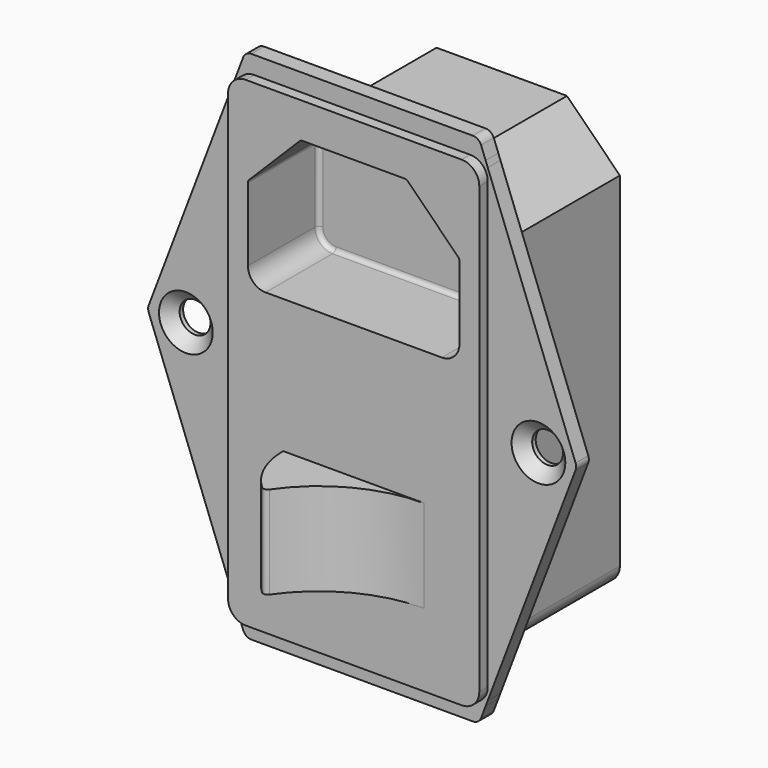
from build123d import *

# Parameters (mm, degrees)
F0_W          = 26.8
F0_H          = 47
F1_DEPTH      = 18
F2_SIZE       = 6
F3_R          = 2
F5_DEPTH      = 5
F6_R          = 1
F7_W          = 28.5
F7_H          = 54.5
F8_DEPTH      = 3
F10_R         = 1.75
F11_DEPTH     = 1.8
F12_T4_DEPTH  = 13
F12_T9_DEPTH  = 13
F12_T14_DEPTH = 13
F12_T19_DEPTH = 13
F12_T24_DEPTH = 13
F12_T29_DEPTH = 13
F12_T34_DEPTH = 13
F12_T39_DEPTH = 13
F13_R         = 1
F14_SIZE      = 1.3
F15_W         = 24
F15_H         = 16.5
F16_DEPTH     = 10
F17_SIZE      = 6
F19_R         = 2
F20_R         = 0.5
F21_W         = 16
F21_H         = 10.5
F22_DEPTH     = 10
F24_DEPTH     = 10.5
F25_R         = 0.5


# Not quite as in the source:
# - a fillet or chamfer that OpenCascade refuses, or shapes differently, is made with other operations: its cross-section is extruded or revolved along the edge and cut away or added


with BuildPart() as f1:
    # F0 (on Front) → F1 (new body)
    with BuildSketch(Plane.XZ):
        Rectangle(F0_W, F0_H)
    extrude(amount=-F1_DEPTH)

    # F2
    f2_edges = [f1.edges().sort_by_distance(p)[0] for p in [
        (-13.4, 9, 23.5),
        (13.4, 9, 23.5),
    ]]
    chamfer(f2_edges, length=F2_SIZE)

    # F3
    f3_edges = [f1.edges().sort_by_distance(p)[0] for p in [
        (-13.4, 9, -23.5),
        (13.4, 9, -23.5),
    ]]
    fillet(f3_edges, radius=F3_R)

    # F4 (on face) → F5 (cut)
    with BuildSketch(Plane(origin=(0, 18, 0), x_dir=(-1, 0, 0), z_dir=(0, 1, 0))):
        Polygon((-6.5715728753, 21.5), (-11.4, 16.6715728753), (-11.4, -21.5), (11.4, -21.5), (11.4, 16.6715728753), (6.5715728753, 21.5), align=None)
    extrude(amount=-F5_DEPTH, mode=Mode.SUBTRACT)

    # F6
    f6_edges = [f1.edges().sort_by_distance(p)[0] for p in [
        (-11.4, 15.5, -21.5),
        (-11.4, 15.5, 16.671573),
        (-6.571573, 15.5, 21.5),
        (6.571573, 15.5, 21.5),
        (11.4, 15.5, 16.671573),
        (11.4, 15.5, -21.5),
        (-8.985786, 13, 19.085786),
        (0, 13, 21.5),
        (8.985786, 13, 19.085786),
        (11.4, 13, -2.414214),
        (0, 13, -21.5),
        (-11.4, 13, -2.414214),
    ]]
    fillet(f6_edges, radius=F6_R)

    # F7 (on face) → F8 (join)
    with BuildSketch(Plane.XZ):
        Rectangle(F7_W, F7_H)
    extrude(amount=F8_DEPTH)

    # F10 (on offset) → F11 (join)
    with BuildSketch(Plane.XZ.offset(1.8)):
        Polygon((24.35, 0), (13.25, 29.25), (-13.25, 29.25), (-24.35, 0), (-13.25, -29.25), (13.25, -29.25), align=None)
        with Locations((-20, 0)):
            Circle(F10_R, mode=Mode.SUBTRACT)
        with Locations((20, 0)):
            Circle(F10_R, mode=Mode.SUBTRACT)
    extrude(amount=-F11_DEPTH)

    # F12: fillet of radius 2 on 4 edges, made by hand


with BuildPart() as f12_tool2:
    # F12_s3 → F12_t4 (new body)
    with BuildSketch(Plane.XZ.offset(-5)):
        with BuildLine():
            ThreePointArc((12.25, 27.25), (13.6642135624, 26.6642135624), (14.25, 25.25))
            Line((14.25, 25.25), (14.25, 27.25))
            Line((14.25, 27.25), (12.25, 27.25))
        make_face()
    extrude(amount=F12_T4_DEPTH)

    split(bisect_by=Plane.XZ.offset(1.8), keep=Keep.TOP)


with BuildPart() as f1_1:
    add(f1.part)

    # F12_t1: cut F12_tool2
    add(f12_tool2.part, mode=Mode.SUBTRACT)


with BuildPart() as f12_tool7:
    # F12_s8 → F12_t9 (new body)
    with BuildSketch(Plane.XZ.offset(-5)):
        with BuildLine():
            ThreePointArc((12.25, 27.25), (13.6642135624, 26.6642135624), (14.25, 25.25))
            Line((14.25, 25.25), (14.25, 27.25))
            Line((14.25, 27.25), (12.25, 27.25))
        make_face()
    extrude(amount=F12_T9_DEPTH)

    split(bisect_by=Plane(origin=(21.2847693156, 0, 8.0772970736), x_dir=(0, 1, 0), z_dir=(0.9349426915, 0, 0.354798765)), keep=Keep.TOP)


with BuildPart() as f1_2:
    add(f1_1.part)

    # F12_t6: cut F12_tool7
    add(f12_tool7.part, mode=Mode.SUBTRACT)


with BuildPart() as f12_tool12:
    # F12_s13 → F12_t14 (new body)
    with BuildSketch(Plane.XZ.offset(-5)):
        with BuildLine():
            ThreePointArc((-12.25, 27.25), (-13.6642135624, 26.6642135624), (-14.25, 25.25))
            Line((-14.25, 25.25), (-14.25, 27.25))
            Line((-14.25, 27.25), (-12.25, 27.25))
        make_face()
    extrude(amount=F12_T14_DEPTH)

    split(bisect_by=Plane.XZ.offset(1.8), keep=Keep.TOP)


with BuildPart() as f1_3:
    add(f1_2.part)

    # F12_t11: cut F12_tool12
    add(f12_tool12.part, mode=Mode.SUBTRACT)


with BuildPart() as f12_tool17:
    # F12_s18 → F12_t19 (new body)
    with BuildSketch(Plane.XZ.offset(-5)):
        with BuildLine():
            ThreePointArc((-12.25, 27.25), (-13.6642135624, 26.6642135624), (-14.25, 25.25))
            Line((-14.25, 25.25), (-14.25, 27.25))
            Line((-14.25, 27.25), (-12.25, 27.25))
        make_face()
    extrude(amount=F12_T19_DEPTH)

    split(bisect_by=Plane(origin=(-21.2847693156, 0, 8.0772970736), x_dir=(0, 1, 0), z_dir=(-0.9349426915, 0, 0.354798765)), keep=Keep.TOP)


with BuildPart() as f1_4:
    add(f1_3.part)

    # F12_t16: cut F12_tool17
    add(f12_tool17.part, mode=Mode.SUBTRACT)


with BuildPart() as f12_tool22:
    # F12_s23 → F12_t24 (new body)
    with BuildSketch(Plane.XZ.offset(-5)):
        with BuildLine():
            ThreePointArc((14.25, -25.25), (13.6642135624, -26.6642135624), (12.25, -27.25))
            Line((12.25, -27.25), (14.25, -27.25))
            Line((14.25, -27.25), (14.25, -25.25))
        make_face()
    extrude(amount=F12_T24_DEPTH)

    split(bisect_by=Plane.XZ.offset(1.8), keep=Keep.TOP)


with BuildPart() as f1_5:
    add(f1_4.part)

    # F12_t21: cut F12_tool22
    add(f12_tool22.part, mode=Mode.SUBTRACT)


with BuildPart() as f12_tool27:
    # F12_s28 → F12_t29 (new body)
    with BuildSketch(Plane.XZ.offset(-5)):
        with BuildLine():
            ThreePointArc((14.25, -25.25), (13.6642135624, -26.6642135624), (12.25, -27.25))
            Line((12.25, -27.25), (14.25, -27.25))
            Line((14.25, -27.25), (14.25, -25.25))
        make_face()
    extrude(amount=F12_T29_DEPTH)

    split(bisect_by=Plane(origin=(21.2847693156, 0, -8.0772970736), x_dir=(0, 1, 0), z_dir=(0.9349426915, 0, -0.354798765)), keep=Keep.TOP)


with BuildPart() as f1_6:
    add(f1_5.part)

    # F12_t26: cut F12_tool27
    add(f12_tool27.part, mode=Mode.SUBTRACT)


with BuildPart() as f12_tool32:
    # F12_s33 → F12_t34 (new body)
    with BuildSketch(Plane.XZ.offset(-5)):
        with BuildLine():
            ThreePointArc((-14.25, -25.25), (-13.6642135624, -26.6642135624), (-12.25, -27.25))
            Line((-12.25, -27.25), (-14.25, -27.25))
            Line((-14.25, -27.25), (-14.25, -25.25))
        make_face()
    extrude(amount=F12_T34_DEPTH)

    split(bisect_by=Plane.XZ.offset(1.8), keep=Keep.TOP)


with BuildPart() as f1_7:
    add(f1_6.part)

    # F12_t31: cut F12_tool32
    add(f12_tool32.part, mode=Mode.SUBTRACT)


with BuildPart() as f12_tool37:
    # F12_s38 → F12_t39 (new body)
    with BuildSketch(Plane.XZ.offset(-5)):
        with BuildLine():
            ThreePointArc((-14.25, -25.25), (-13.6642135624, -26.6642135624), (-12.25, -27.25))
            Line((-12.25, -27.25), (-14.25, -27.25))
            Line((-14.25, -27.25), (-14.25, -25.25))
        make_face()
    extrude(amount=F12_T39_DEPTH)

    split(bisect_by=Plane(origin=(-21.2847693156, 0, -8.0772970736), x_dir=(0, 1, 0), z_dir=(-0.9349426915, 0, -0.354798765)), keep=Keep.TOP)


with BuildPart() as f1_8:
    add(f1_7.part)

    # F12_t36: cut F12_tool37
    add(f12_tool37.part, mode=Mode.SUBTRACT)

    # F13
    f13_edges = [f1_8.edges().sort_by_distance(p)[0] for p in [
        (-13.25, -0.9, 29.25),
        (13.25, -0.9, 29.25),
        (-24.35, -0.9, 0),
        (-13.25, -0.9, -29.25),
        (13.25, -0.9, -29.25),
        (24.35, -0.9, 0),
    ]]
    fillet(f13_edges, radius=F13_R)

    # F14
    f14_edges = [f1_8.edges().sort_by_distance(p)[0] for p in [
        (-21.75, -1.8, 0),
        (18.25, -1.8, 0),
    ]]
    chamfer(f14_edges, length=F14_SIZE)


with BuildPart() as f16:
    # F15 (on face) → F16 (new body)
    with BuildSketch(Plane.XZ.offset(3)):
        with Locations((0, 15)):
            Rectangle(F15_W, F15_H)
    extrude(amount=-F16_DEPTH)

    # F17
    f17_edges = [f16.edges().sort_by_distance(p)[0] for p in [
        (12, 2, 23.25),
        (-12, 2, 23.25),
    ]]
    chamfer(f17_edges, length=F17_SIZE)


with BuildPart() as f1_9:
    add(f1_8.part)

    # F18: cut F16
    add(f16.part, mode=Mode.SUBTRACT)

    # F19
    f19_edges = [f1_9.edges().sort_by_distance(p)[0] for p in [
        (-12, 2, 6.75),
        (12, 2, 6.75),
    ]]
    fillet(f19_edges, radius=F19_R)

    # F20
    f20_edges = [f1_9.edges().sort_by_distance(p)[0] for p in [
        (12, 2, 17.25),
        (6, 2, 23.25),
        (-12, 2, 17.25),
        (-6, 2, 23.25),
        (12, 7, 13),
        (11.414214, 7, 7.335786),
        (9, 7, 20.25),
        (0, 7, 6.75),
        (0, 7, 23.25),
        (-11.414214, 7, 7.335786),
        (-9, 7, 20.25),
        (-12, 7, 13),
    ]]
    fillet(f20_edges, radius=F20_R)

    # F21 (on face) → F22 (cut)
    with BuildSketch(Plane.XZ.offset(3)):
        with Locations((0, -13.7)):
            Rectangle(F21_W, F21_H)
    extrude(amount=-F22_DEPTH, mode=Mode.SUBTRACT)

    # F23 (on face) → F24 (join, through all)
    with BuildSketch(Plane.XY.offset(-18.95)):
        with BuildLine():
            ThreePointArc((-4.6646603483, -9.9856908622), (0.7682384829, -4.8622275452), (8, -3))
            Line((8, -3), (8, -1.4239461161))
            Line((8, -1.4239461161), (-8, -1.4239461161))
            Line((-8, -1.4239461161), (-8, -3))
            ThreePointArc((-8, -3), (-7.1233945241, -6.8705415453), (-4.6646603483, -9.9856908622))
        make_face()
    extrude(amount=F24_DEPTH)

    # F25
    f25_edges = [f1_9.edges().sort_by_distance(p)[0] for p in [
        (-4.66466, -9.985691, -13.7),
    ]]
    fillet(f25_edges, radius=F25_R)


solid = f1_9.part
